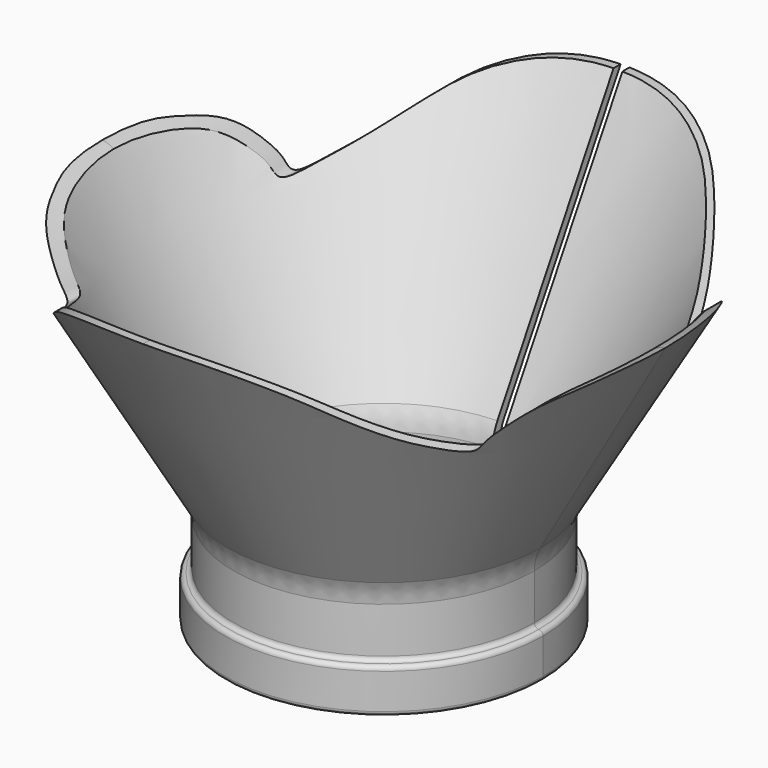
from build123d import *

# Parameters (mm, degrees)
F0_R          = 17
F0_R_2        = 16
F1_DEPTH      = 12
F2_W          = 1
F2_H          = 5
F5_DEPTH      = 34.3215080757
F5_DEPTH_BACK = 34.3215080757
F6_W          = 1
F6_H          = 50
F7_DEPTH      = 41.5955775602
F8_R          = 5
F9_R          = 5
F10_R         = 0.49999


# Not quite as in the source:
# - a fillet or chamfer is up to 0.001 mm smaller than in the source, because OpenCascade refuses the exact size


with BuildPart() as f1:
    # F0 (on Top) → F1 (new body)
    with BuildSketch(Plane.XY):
        Circle(F0_R)
        Circle(F0_R_2, mode=Mode.SUBTRACT)
    extrude(amount=F1_DEPTH)

    # F2 (on Front) → F3 (revolve)
    with BuildSketch(Plane.XZ):
        Polygon((16, 12), (17, 12), (34.3205080757, 42), (33.5705080757, 42.4330127019), align=None)
        with Locations((17.5, 2.5)):
            Rectangle(F2_W, F2_H)
    revolve(axis=Axis((0, 0, 30.9658702463), (0, 0, 1)))

    # F4 (on Front) → F5 (cut, two sides)
    with BuildSketch(Plane.XZ) as f5_sk:
        with BuildLine():
            Line((60, 60.1254698044), (-60, 60.1254698044))
            Line((-60, 60.1254698044), (-60, 27))
            Line((-60, 27), (-45.7045286894, 27))
            add(Edge.make_bspline(
                [(0, 41.5941886604), (-2.8405018148, 41.6049536738), (-7.4476144034, 41.211227315), (-12.9991792451, 39.1055660324), (-16.0905576066, 36.442538994), (-19.3952617181, 33.3207316284), (-21.3663159983, 31.9181584991), (-22.9486655756, 30.6397166663), (-23.9236337156, 32.2233697002), (-25.6640615728, 33.9410144278), (-28.0740492048, 36.118739208), (-30.562257894, 37.1637389425), (-33.4042561904, 38.9158578145), (-42.4905985298, 31.1136082335), (-45.7045286894, 27)],
                knots=[0, 0, 0, 0, 0.1152973029, 0.2141555908, 0.2988270346, 0.3869286449, 0.4536574145, 0.5054448357, 0.5549660833, 0.6217164901, 0.6970517629, 0.7642831784, 0.8303982296, 1, 1, 1, 1], degree=3))
            add(Edge.make_bspline(
                [(0, 41.5941886604), (2.8405018148, 41.6049536738), (7.4476144034, 41.211227315), (12.9991792451, 39.1055660324), (16.0905576066, 36.442538994), (19.3952617181, 33.3207316284), (21.3663159983, 31.9181584991), (22.9486655756, 30.6397166663), (23.9236337156, 32.2233697002), (25.6640615728, 33.9410144278), (28.0740492048, 36.118739208), (30.562257894, 37.1637389425), (33.4042561904, 38.9158578145), (42.4905985298, 31.1136082335), (45.7045286894, 27)],
                knots=[0, 0, 0, 0, 0.1152973029, 0.2141555908, 0.2988270346, 0.3869286449, 0.4536574145, 0.5054448357, 0.5549660833, 0.6217164901, 0.6970517629, 0.7642831784, 0.8303982296, 1, 1, 1, 1], degree=3))
            Line((45.7045286894, 27), (60, 27))
            Line((60, 27), (60, 60.1254698044))
        make_face()
    extrude(amount=-F5_DEPTH, mode=Mode.SUBTRACT)
    extrude(f5_sk.sketch, amount=F5_DEPTH_BACK, mode=Mode.SUBTRACT)

    # F6 (on Top) → F7 (cut, through all)
    with BuildSketch(Plane.XY):
        with Locations((0, 25)):
            Rectangle(F6_W, F6_H)
    extrude(amount=F7_DEPTH, mode=Mode.SUBTRACT)

    # F8
    f8_edges = [f1.edges().sort_by_distance(p)[0] for p in [
        (-11.135529, -11.489125, 12),
        (11.489125, 11.135529, 12),
    ]]
    fillet(f8_edges, radius=F8_R)

    # F9
    f9_edges = [f1.edges().sort_by_distance(p)[0] for p in [
        (-11.842719, -12.196311, 12),
        (12.196311, 11.842719, 12),
    ]]
    fillet(f9_edges, radius=F9_R)

    # F10 (radius 0.5 in the source; OpenCascade refuses exactly that, so slightly less here)
    f10_edges = [f1.edges().sort_by_distance(p)[0] for p in [
        (-11.842719, -12.196311, 5),
        (12.196311, 11.842719, 5),
        (-12.5499, -12.903488, 5),
        (12.903488, 12.5499, 5),
        (-11.135529, -11.489125, 0),
        (12.903488, 12.5499, 0),
        (-12.5499, -12.903488, 0),
    ]]
    fillet(f10_edges, radius=F10_R)


solid = f1.part
